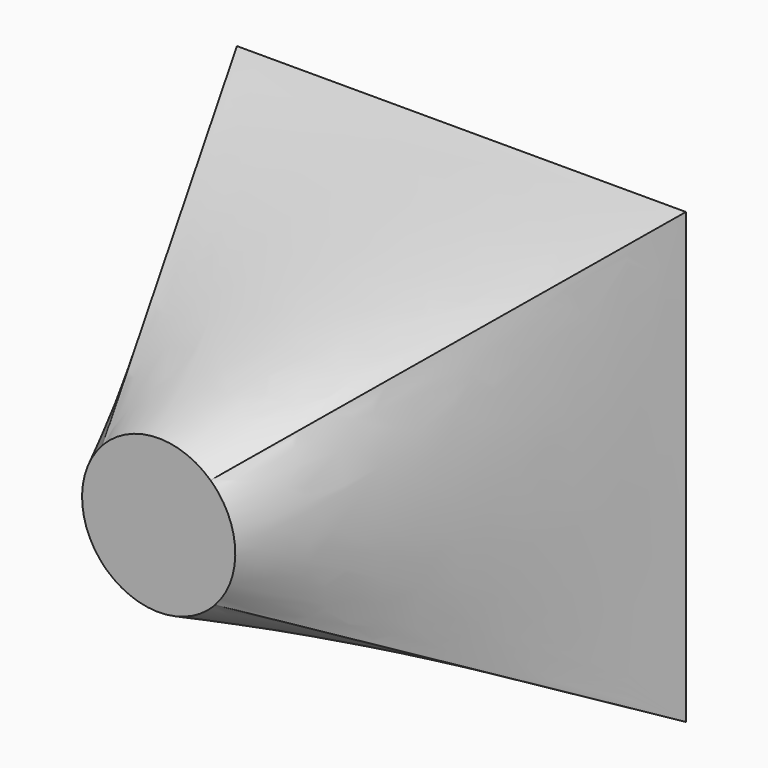
from build123d import *

# Parameters (mm, degrees)
F0_W = 101.6
F0_H = 101.6


# Not quite as in the source:
# - the arcs of a loft's sections are written as splines that run evenly, so that the points pair up as in the source's solid


with BuildPart() as f3:
    # F2 (on offset) → F3 section 0
    with BuildSketch(Plane.XZ.offset(83.82)):
        with BuildLine():
            add(Edge.make_bspline(
                [(-12.7675348715, 11.7290260492), (-13.5351978313, 10.893392846), (-14.2205411574, 9.9821739727), (-15.4003183185, 8.0434932535), (-15.8947229813, 7.0160793452), (-16.6736132092, 4.8844867261), (-16.9580795149, 3.7803607232), (-17.3061504951, 1.5377721132), (-17.3697465629, 0.3993649586), (-17.2736221227, -1.8680382197), (-17.1139039916, -2.9969781774), (-16.5772781394, -5.2020608915), (-16.2003836875, -6.2781491228), (-15.2438786538, -8.3361712805), (-14.6642917235, -9.3180543182), (-13.3246654604, -11.1499272821), (-12.5646592525, -11.9998719117), (-11.7290260492, -12.7675348715)],
                knots=[0, 0, 0, 0, 0.125, 0.125, 0.25, 0.25, 0.375, 0.375, 0.5, 0.5, 0.625, 0.625, 0.75, 0.75, 0.875, 0.875, 1, 1, 1, 1], degree=3))
            add(Edge.make_bspline(
                [(-11.7290260492, -12.7675348715), (-10.893392846, -13.5351978313), (-9.9821739727, -14.2205411574), (-8.0434932535, -15.4003183185), (-7.0160793452, -15.8947229813), (-4.8844867261, -16.6736132092), (-3.7803607232, -16.9580795149), (-1.5377721132, -17.3061504951), (-0.3993649586, -17.3697465629), (1.8680382197, -17.2736221227), (2.9969781774, -17.1139039916), (5.2020608915, -16.5772781394), (6.2781491228, -16.2003836875), (8.3361712805, -15.2438786538), (9.3180543182, -14.6642917235), (11.1499272821, -13.3246654604), (11.9998719117, -12.5646592525), (12.7675348715, -11.7290260492)],
                knots=[0, 0, 0, 0, 0.125, 0.125, 0.25, 0.25, 0.375, 0.375, 0.5, 0.5, 0.625, 0.625, 0.75, 0.75, 0.875, 0.875, 1, 1, 1, 1], degree=3))
            add(Edge.make_bspline(
                [(12.7675348715, -11.7290260492), (13.5351978313, -10.893392846), (14.2205411574, -9.9821739727), (15.4003183185, -8.0434932535), (15.8947229813, -7.0160793452), (16.6736132092, -4.8844867261), (16.9580795149, -3.7803607232), (17.3061504951, -1.5377721132), (17.3697465629, -0.3993649586), (17.2736221227, 1.8680382197), (17.1139039916, 2.9969781774), (16.5772781394, 5.2020608915), (16.2003836875, 6.2781491228), (15.2438786538, 8.3361712805), (14.6642917235, 9.3180543182), (13.3246654604, 11.1499272821), (12.5646592525, 11.9998719117), (11.7290260492, 12.7675348715)],
                knots=[0, 0, 0, 0, 0.125, 0.125, 0.25, 0.25, 0.375, 0.375, 0.5, 0.5, 0.625, 0.625, 0.75, 0.75, 0.875, 0.875, 1, 1, 1, 1], degree=3))
            add(Edge.make_bspline(
                [(11.7290260492, 12.7675348715), (10.893392846, 13.5351978313), (9.9821739727, 14.2205411574), (8.0434932535, 15.4003183185), (7.0160793452, 15.8947229813), (4.8844867261, 16.6736132092), (3.7803607232, 16.9580795149), (1.5377721132, 17.3061504951), (0.3993649586, 17.3697465629), (-1.8680382197, 17.2736221227), (-2.9969781774, 17.1139039916), (-5.2020608915, 16.5772781394), (-6.2781491228, 16.2003836875), (-8.3361712805, 15.2438786538), (-9.3180543182, 14.6642917235), (-11.1499272821, 13.3246654604), (-11.9998719117, 12.5646592525), (-12.7675348715, 11.7290260492)],
                knots=[0, 0, 0, 0, 0.125, 0.125, 0.25, 0.25, 0.375, 0.375, 0.5, 0.5, 0.625, 0.625, 0.75, 0.75, 0.875, 0.875, 1, 1, 1, 1], degree=3))
        make_face()
    # F0 (on Front) → F3 section 1
    with BuildSketch(Plane.XZ):
        with Locations((1.4547277242, -5.4684626475)):
            Rectangle(F0_W, F0_H)
    loft(ruled=True)


solid = f3.part
